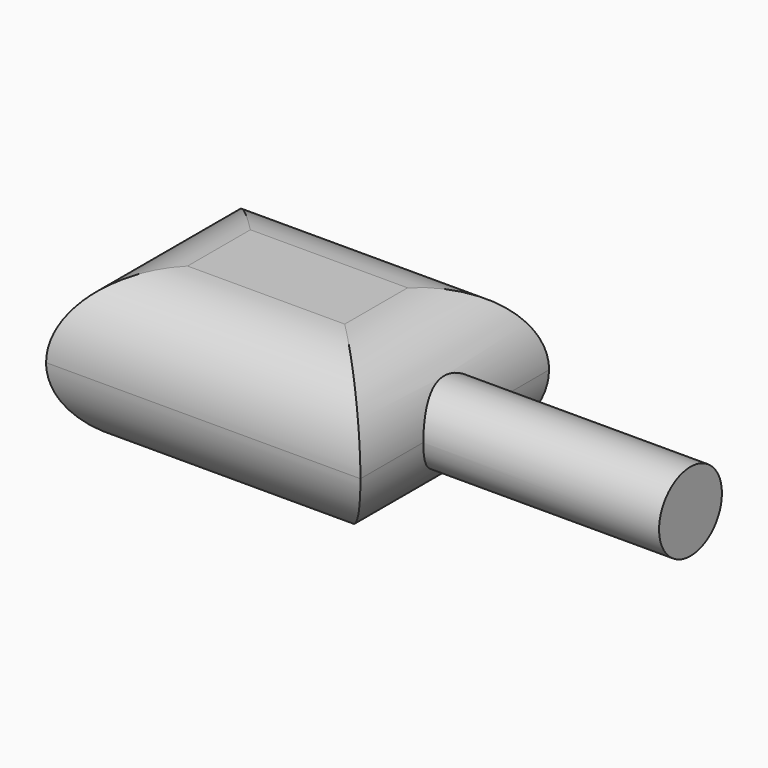
from build123d import *

# Parameters (mm, degrees)
F0_W     = 20
F0_H     = 15
F1_DEPTH = 5
F2_R     = 4.99999
F3_R     = 2.5
F4_DEPTH = 25


# Not quite as in the source:
# - a fillet or chamfer is up to 0.001 mm smaller than in the source, because OpenCascade refuses the exact size


with BuildPart() as f1:
    # F0 (on Top) → F1 (new body, symmetric)
    with BuildSketch(Plane.XY):
        Rectangle(F0_W, F0_H)
    extrude(amount=F1_DEPTH, both=True)

    # F2 (radius 5 in the source; OpenCascade refuses exactly that, so slightly less here)
    f2_edges = [f1.edges().sort_by_distance(p)[0] for p in [
        (0, 7.5, 5),
        (-10, 0, 5),
        (0, -7.5, 5),
        (10, 0, 5),
        (0, -7.5, -5),
        (10, 0, -5),
        (0, 7.5, -5),
        (-10, 0, -5),
    ]]
    fillet(f2_edges, radius=F2_R)

    # F3 (on Right) → F4 (join)
    with BuildSketch(Plane.YZ):
        Circle(F3_R)
    extrude(amount=F4_DEPTH)


solid = f1.part
